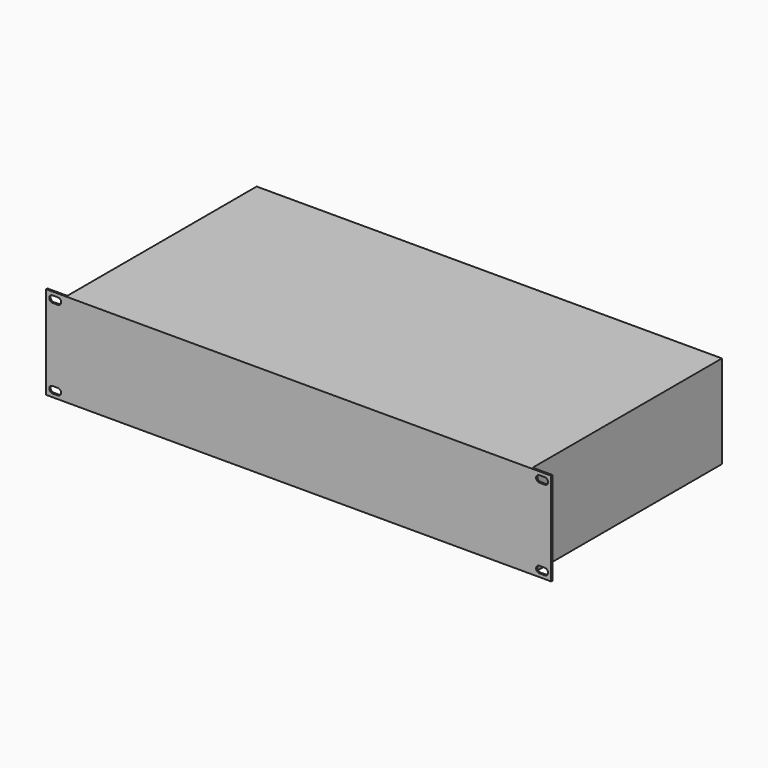
from build123d import *

# Parameters (mm, degrees)
F1_W     = 482.6
F1_H     = 88.9
F2_DEPTH = 1.5875
F3_W     = 444.5
F3_H     = 88.9
F4_DEPTH = 226.06


# Not quite as in the source:
# - a variable given as a bare number and used for a length is read in inches; the dataset says mm whatever the document's units were


with BuildPart() as f2:
    # F1 (on Front) → F2 (new body)
    with BuildSketch(Plane.XZ):
        Rectangle(F1_W, F1_H)
        with BuildLine():
            Line((-235.1024, -34.925), (-230.0224, -34.925))
            ThreePointArc((-230.0224, -34.925), (-226.8474, -38.1), (-230.0224, -41.275))
            Line((-230.0224, -41.275), (-235.1024, -41.275))
            ThreePointArc((-235.1024, -41.275), (-238.2774, -38.1), (-235.1024, -34.925))
        make_face(mode=Mode.SUBTRACT)
        with BuildLine():
            Line((230.0224, -34.925), (235.1024, -34.925))
            ThreePointArc((235.1024, -34.925), (238.2774, -38.1), (235.1024, -41.275))
            Line((235.1024, -41.275), (230.0224, -41.275))
            ThreePointArc((230.0224, -41.275), (226.8474, -38.1), (230.0224, -34.925))
        make_face(mode=Mode.SUBTRACT)
        with BuildLine():
            ThreePointArc((-235.1024, 34.925), (-238.2774, 38.1), (-235.1024, 41.275))
            Line((-235.1024, 41.275), (-230.0224, 41.275))
            ThreePointArc((-230.0224, 41.275), (-226.8474, 38.1), (-230.0224, 34.925))
            Line((-230.0224, 34.925), (-235.1024, 34.925))
        make_face(mode=Mode.SUBTRACT)
        with BuildLine():
            Line((235.1024, 34.925), (230.0224, 34.925))
            ThreePointArc((230.0224, 34.925), (226.8474, 38.1), (230.0224, 41.275))
            Line((230.0224, 41.275), (235.1024, 41.275))
            ThreePointArc((235.1024, 41.275), (238.2774, 38.1), (235.1024, 34.925))
        make_face(mode=Mode.SUBTRACT)
    extrude(amount=F2_DEPTH)

    # F3 (on face) → F4 (join)
    with BuildSketch(Plane(origin=(0, 0, 0), x_dir=(-1, 0, 0), z_dir=(0, 1, 0))):
        Rectangle(F3_W, F3_H)
    extrude(amount=F4_DEPTH)


solid = f2.part
